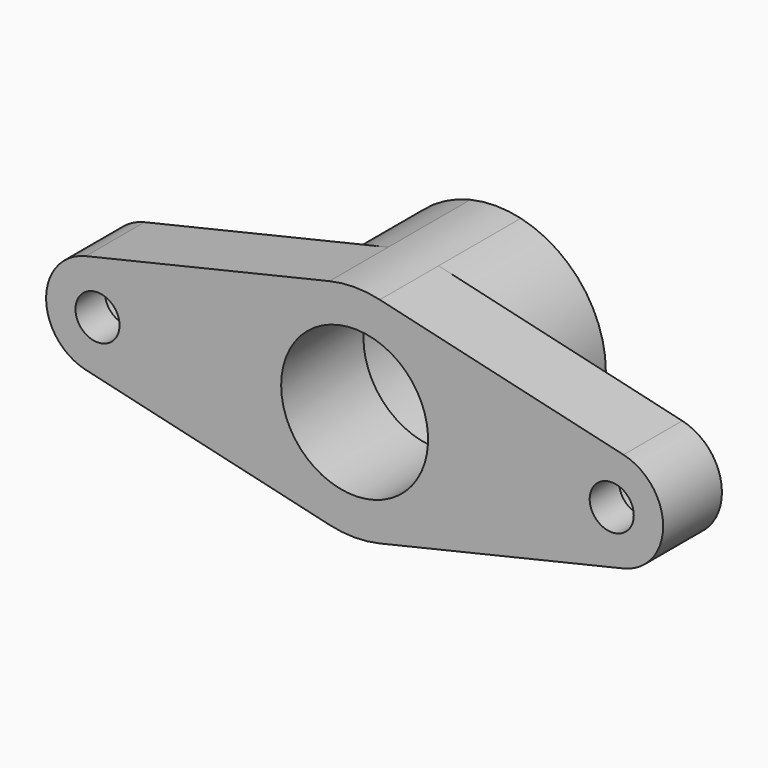
from build123d import *

# Parameters (mm, degrees)
F1_DEPTH  = 10
F2_R      = 3
F3_DEPTH  = 10
F4_R      = 4.5
F4_R_2    = 3
F5_DEPTH  = 5
F6_R      = 4.5
F7_DEPTH  = 5
F8_DEPTH  = 5
F10_DEPTH = 14
F11_R     = 10
F12_DEPTH = 20
F13_R     = 10
F14_DEPTH = 40
F15_R     = 12
F15_R_2   = 10
F16_DEPTH = 10


with BuildPart() as f1:
    # F0 (on Front) → F1 (new body)
    with BuildSketch(Plane.XZ):
        with BuildLine():
            Line((32.1521708727, 21.1400806223), (-1.0192576987, 28.9282977823))
            ThreePointArc((-1.0192576987, 28.9282977823), (-4.4478291273, 29.3253906074), (-7.8764005559, 28.9282977823))
            Line((-7.8764005559, 28.9282977823), (-41.0478291273, 21.1400806223))
            ThreePointArc((-41.0478291273, 21.1400806223), (-46.4478291273, 14.3253906074), (-41.0478291273, 7.5107005924))
            Line((-41.0478291273, 7.5107005924), (-7.8764005559, -0.2775165675))
            ThreePointArc((-7.8764005559, -0.2775165675), (-4.4478291273, -0.6746093926), (-1.0192576987, -0.2775165675))
            Line((-1.0192576987, -0.2775165675), (32.1521708727, 7.5107005924))
            ThreePointArc((32.1521708727, 7.5107005924), (37.5521708727, 14.3253906074), (32.1521708727, 21.1400806223))
        make_face()
    extrude(amount=F1_DEPTH)

    # F2 (on face) → F3 (cut)
    with BuildSketch(Plane.XZ.offset(10)):
        with Locations((-39.4478291273, 14.3253906074)):
            Circle(F2_R)
        with Locations((30.5521708727, 14.3253906074)):
            Circle(F2_R)
    extrude(amount=-F3_DEPTH, mode=Mode.SUBTRACT)

    # F4 (on face) → F5 (join)
    with BuildSketch(Plane.XZ.offset(10)):
        with Locations((-39.4478291273, 14.3253906074)):
            Circle(F4_R)
        with Locations((-39.4478291273, 14.3253906074)):
            Circle(F4_R_2, mode=Mode.SUBTRACT)
        with Locations((30.5521708727, 14.3253906074)):
            Circle(F4_R)
        with Locations((30.5521708727, 14.3253906074)):
            Circle(F4_R_2, mode=Mode.SUBTRACT)
    extrude(amount=-F5_DEPTH)

    # F6 (on Front) → F7 (cut)
    with BuildSketch(Plane.XZ):
        with Locations((-39.4478291273, 14.3253906074)):
            Circle(F6_R)
    extrude(amount=-F7_DEPTH, mode=Mode.SUBTRACT)

    # F6 (on Front) → F8 (cut)
    with BuildSketch(Plane.XZ):
        with Locations((-39.4478291273, 14.3253906074)):
            Circle(F6_R)
        with Locations((30.5521708727, 14.3253906074)):
            Circle(F6_R)
    extrude(amount=F8_DEPTH, mode=Mode.SUBTRACT)

    # F9 (on face) → F10 (join)
    with BuildSketch(Plane(origin=(0, 0, 0), x_dir=(-1, 0, 0), z_dir=(0, 1, 0))):
        with BuildLine():
            ThreePointArc((7.8764005559, -0.2775165675), (16.2042863196, 5.0095055563), (19.4478291273, 14.3253906074))
            ThreePointArc((19.4478291273, 14.3253906074), (16.2042863196, 23.6412756585), (7.8764005559, 28.9282977823))
            ThreePointArc((7.8764005559, 28.9282977823), (4.4478291273, 29.3253906074), (1.0192576987, 28.9282977823))
            ThreePointArc((1.0192576987, 28.9282977823), (-10.5521708727, 14.3253906074), (1.0192576987, -0.2775165675))
            ThreePointArc((1.0192576987, -0.2775165675), (4.4478291273, -0.6746093926), (7.8764005559, -0.2775165675))
        make_face()
    extrude(amount=F10_DEPTH)

    # F11 (on face) → F12 (cut)
    with BuildSketch(Plane(origin=(0, 14, 0), x_dir=(-1, 0, 0), z_dir=(0, 1, 0))):
        with Locations((4.4478291273, 14.3253906074)):
            Circle(F11_R)
    extrude(amount=F12_DEPTH, mode=Mode.SUBTRACT)

    # F13 (on face) → F14 (cut)
    with BuildSketch(Plane(origin=(0, 14, 0), x_dir=(-1, 0, 0), z_dir=(0, 1, 0))):
        with Locations((4.4478291273, 14.3253906074)):
            Circle(F13_R)
    extrude(amount=-F14_DEPTH, mode=Mode.SUBTRACT)

    # F15 (on face) → F16 (cut)
    with BuildSketch(Plane(origin=(0, 14, 0), x_dir=(-1, 0, 0), z_dir=(0, 1, 0))):
        with Locations((4.4478291273, 14.3253906074)):
            Circle(F15_R)
        with Locations((4.4478291273, 14.3253906074)):
            Circle(F15_R_2, mode=Mode.SUBTRACT)
    extrude(amount=-F16_DEPTH, mode=Mode.SUBTRACT)


solid = f1.part
